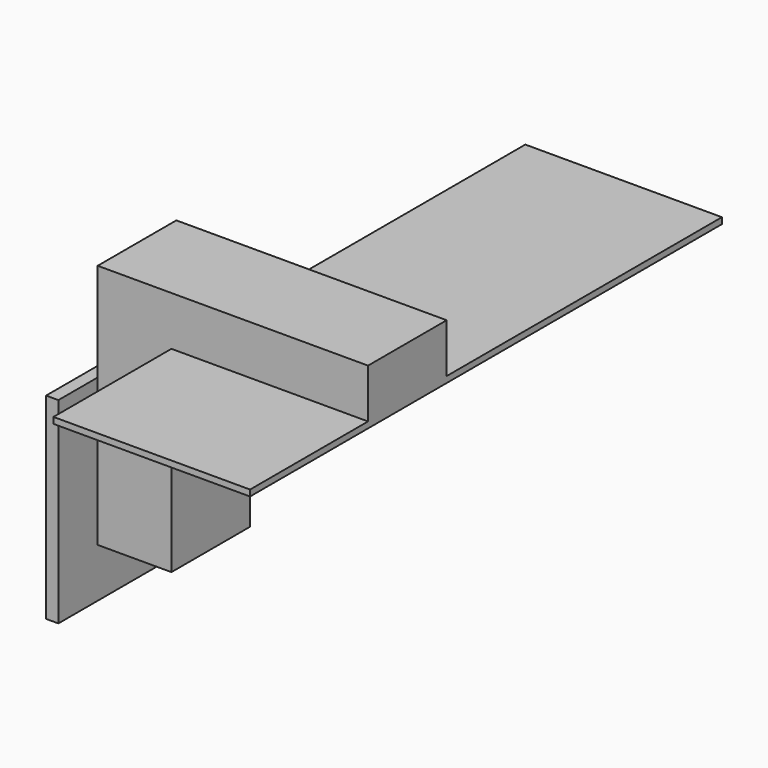
from build123d import *

# Parameters (mm, degrees)
F0_W     = 101.6
F0_H     = 304.8
F1_DEPTH = 3.175
F2_W     = 38.1
F2_H     = 50.8
F2_W_2   = 101.6
F3_DEPTH = 25.4
F4_DEPTH = 101.6
F6_DEPTH = 6.35


# Not quite as in the source:
# - the program builds the solid bodies; features that only make, move or delete a surface that nothing else refers to are left out


with BuildPart() as f1:
    # F0 (on Top) → F1 (new body)
    with BuildSketch(Plane.XY):
        with Locations((17.6723517966, 8.8070686907)):
            Rectangle(F0_W, F0_H)
    extrude(amount=F1_DEPTH)

    # F2 (on face) → F3 (join)
    with BuildSketch(Plane.XY.offset(3.175)):
        with Locations((-52.1776482034, -41.9929313093)):
            Rectangle(F2_W, F2_H)
        with Locations((17.6723517966, -41.9929313093)):
            Rectangle(F2_W_2, F2_H)
    extrude(amount=F3_DEPTH)

    # F4 (add): a face of the model
    f4_faces = [f1.faces().sort_by_distance(p)[0] for p in [
        (-52.1776482034, -41.9929313093, 3.175),
    ]]
    extrude(f4_faces, amount=F4_DEPTH)

    # F5 (on face) → F6 (join)
    with BuildSketch(Plane(origin=(-71.2276482034, 0, 0), x_dir=(0, -1, 0), z_dir=(-1, 0, 0))):
        Polygon((92.7929313093, -123.825), (92.7929313093, -22.225), (67.3929313093, -22.225), (67.3929313093, -98.425), (41.9929313093, -98.425), (16.5929313093, -98.425), (16.5929313093, -22.225), (-8.8070686907, -22.225), (-8.8070686907, -123.825), align=None)
        Polygon((67.3929313093, -98.425), (67.3929313093, -22.225), (16.5929313093, -22.225), (16.5929313093, -98.425), (41.9929313093, -98.425), align=None)
    extrude(amount=F6_DEPTH)


solid = f1.part
